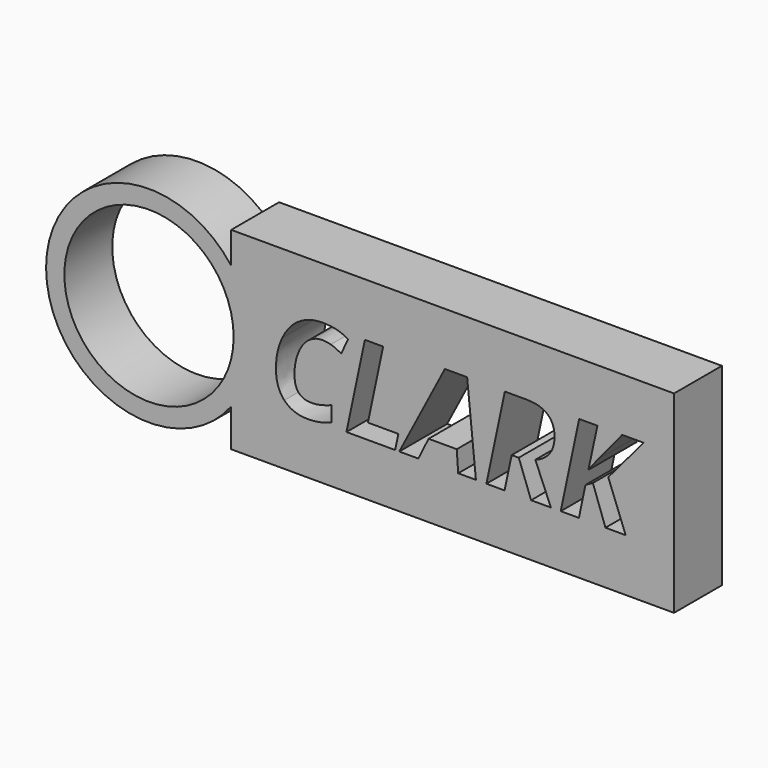
from build123d import *

# Parameters (mm, degrees)
F0_R     = 35.3591127091
F1_DEPTH = 25


with BuildPart() as f1:
    # F0 (on Front) → F1 (new body)
    with BuildSketch(Plane.XZ):
        with BuildLine():
            Line((61.9367249054, 34.8669122506), (-123.0632750946, 34.8669122506))
            Line((-123.0632750946, 34.8669122506), (-123.0632750946, 21.6819903858))
            ThreePointArc((-123.0632750946, 21.6819903858), (-116.6274794012, 9.4492653106), (-114.4056740389, -4.193410743))
            ThreePointArc((-114.4056740389, -4.193410743), (-116.6274794012, -17.8360867967), (-123.0632750946, -30.0688118719))
            Line((-123.0632750946, -30.0688118719), (-123.0632750946, -45.8291395163))
            Line((-123.0632750946, -45.8291395163), (61.9367249054, -45.8291395163))
            Line((61.9367249054, -45.8291395163), (61.9367249054, 34.8669122506))
        make_face()
        with BuildLine():
            add(Edge.make_bspline(
                [(-81.4851504642, 6.2619487625), (-83.2026240645, 6.7321619524), (-84.9001733771, 6.7321619524)],
                knots=[0, 0, 0, 1, 1, 1], degree=2))
            add(Edge.make_bspline(
                [(-84.9001733771, 6.7321619524), (-88.1836959912, 6.7321619524), (-90.8137019684, 4.7158240365)],
                knots=[0, 0, 0, 1, 1, 1], degree=2))
            add(Edge.make_bspline(
                [(-90.8137019684, 4.7158240365), (-93.4437079457, 2.6994861206), (-95.0376509623, -1.2216137001)],
                knots=[0, 0, 0, 1, 1, 1], degree=2))
            add(Edge.make_bspline(
                [(-95.0376509623, -1.2216137001), (-96.6315939788, -5.1427135208), (-96.6315939788, -9.6535722576)],
                knots=[0, 0, 0, 1, 1, 1], degree=2))
            add(Edge.make_bspline(
                [(-96.6315939788, -9.6535722576), (-96.6315939788, -13.8137635308), (-94.9260749511, -15.8301014467)],
                knots=[0, 0, 0, 1, 1, 1], degree=2))
            add(Edge.make_bspline(
                [(-94.9260749511, -15.8301014467), (-93.2205559234, -17.8464393626), (-89.4827595496, -17.8464393626)],
                knots=[0, 0, 0, 1, 1, 1], degree=2))
            add(Edge.make_bspline(
                [(-89.4827595496, -17.8464393626), (-85.8485694719, -17.8464393626), (-81.0667404223, -15.9257380277)],
                knots=[0, 0, 0, 1, 1, 1], degree=2))
            Line((-81.0667404223, -15.9257380277), (-81.0667404223, -22.4051163899))
            add(Edge.make_bspline(
                [(-81.0667404223, -22.4051163899), (-86.0159334887, -24.3258177248), (-91.0288842757, -24.3258177248)],
                knots=[0, 0, 0, 1, 1, 1], degree=2))
            add(Edge.make_bspline(
                [(-91.0288842757, -24.3258177248), (-97.3488683362, -24.3258177248), (-100.8635126877, -20.5999759237)],
                knots=[0, 0, 0, 1, 1, 1], degree=2))
            add(Edge.make_bspline(
                [(-100.8635126877, -20.5999759237), (-104.3781570392, -16.8741341225), (-104.3781570392, -10.0520580117)],
                knots=[0, 0, 0, 1, 1, 1], degree=2))
            add(Edge.make_bspline(
                [(-104.3781570392, -10.0520580117), (-104.3781570392, -3.524861359), (-101.7879996373, 1.9662723329)],
                knots=[0, 0, 0, 1, 1, 1], degree=2))
            add(Edge.make_bspline(
                [(-101.7879996373, 1.9662723329), (-99.1978422354, 7.4574060249), (-94.8623172304, 10.3105640245)],
                knots=[0, 0, 0, 1, 1, 1], degree=2))
            add(Edge.make_bspline(
                [(-94.8623172304, 10.3105640245), (-90.5267922255, 13.1637220241), (-84.9001733771, 13.1637220241)],
                knots=[0, 0, 0, 1, 1, 1], degree=2))
            add(Edge.make_bspline(
                [(-84.9001733771, 13.1637220241), (-81.7840147798, 13.1637220241), (-79.3691911097, 12.6018571108)],
                knots=[0, 0, 0, 1, 1, 1], degree=2))
            add(Edge.make_bspline(
                [(-79.3691911097, 12.6018571108), (-76.9543674396, 12.0399921975), (-74.188876306, 10.549655477)],
                knots=[0, 0, 0, 1, 1, 1], degree=2))
            Line((-74.188876306, 10.549655477), (-77.1297011715, 4.3173382823))
            add(Edge.make_bspline(
                [(-77.1297011715, 4.3173382823), (-79.7676768638, 5.7917355726), (-81.4851504642, 6.2619487625)],
                knots=[0, 0, 0, 1, 1, 1], degree=2))
        make_face(mode=Mode.SUBTRACT)
        Polygon((-54.5594680573, -23.8237256746), (-74.9061506634, -23.8237256746), (-67.2153756086, 12.5899025382), (-59.5883582745, 12.5899025382), (-65.9641303406, -17.4479536085), (-53.2125862083, -17.4479536085), align=None, mode=Mode.SUBTRACT)
        Polygon((-28.2354991392, -23.8237256746), (-28.8332277704, -15.1526756647), (-40.6124666626, -15.1526756647), (-44.892203662, -23.8237256746), (-52.8619187447, -23.8237256746), (-33.7903905518, 12.7413271247), (-24.4977027654, 12.7413271247), (-20.8396035425, -23.8237256746), align=None, mode=Mode.SUBTRACT)
        with BuildLine():
            Line((-2.9236840366, -9.8528151347), (-5.8884180473, -9.8528151347))
            Line((-5.8884180473, -9.8528151347), (-8.8531520581, -23.8237256746))
            Line((-8.8531520581, -23.8237256746), (-16.4482905319, -23.8237256746))
            Line((-16.4482905319, -23.8237256746), (-8.7575154771, 12.5899025382))
            Line((-8.7575154771, 12.5899025382), (0.1845048457, 12.5899025382))
            add(Edge.make_bspline(
                [(0.1845048457, 12.5899025382), (6.0900637219, 12.5899025382), (9.0547977327, 10.0475634268)],
                knots=[0, 0, 0, 1, 1, 1], degree=2))
            add(Edge.make_bspline(
                [(9.0547977327, 10.0475634268), (12.0195317435, 7.5052243154), (12.0195317435, 2.6038495396)],
                knots=[0, 0, 0, 1, 1, 1], degree=2))
            add(Edge.make_bspline(
                [(12.0195317435, 2.6038495396), (12.0195317435, -1.3331897113), (9.9513906795, -4.1584537081)],
                knots=[0, 0, 0, 1, 1, 1], degree=2))
            add(Edge.make_bspline(
                [(9.9513906795, -4.1584537081), (7.8832496155, -6.9837177049), (3.9940286552, -8.3545086991)],
                knots=[0, 0, 0, 1, 1, 1], degree=2))
            Line((3.9940286552, -8.3545086991), (10.4973161627, -23.8237256746))
            Line((10.4973161627, -23.8237256746), (2.2247519068, -23.8237256746))
            Line((2.2247519068, -23.8237256746), (-2.9236840366, -9.8528151347))
        make_face(mode=Mode.SUBTRACT)
        Polygon((34.4542797012, -4.8478340628), (41.7067204265, -23.8237256746), (33.2827315841, -23.8237256746), (28.0306893446, -9.0797527717), (24.9145307472, -10.8251203748), (22.2048276191, -23.8237256746), (14.6096891453, -23.8237256746), (22.3004642001, 12.5899025382), (29.9274815343, 12.5899025382), (26.14186687, -4.8956523532), (30.0709364057, 0.2129350148), (40.2562322814, 12.5899025382), (49.2540406098, 12.5899025382), align=None, mode=Mode.SUBTRACT)
        with BuildLine():
            ThreePointArc((-114.4056740389, -4.193410743), (-116.6274794012, 9.4492653106), (-123.0632750946, 21.6819903858))
            ThreePointArc((-123.0632750946, 21.6819903858), (-200.3983681841, -4.193410743), (-123.0632750946, -30.0688118719))
            ThreePointArc((-123.0632750946, -30.0688118719), (-116.6274794012, -17.8360867967), (-114.4056740389, -4.193410743))
        make_face()
        with Locations((-157.4020211115, -4.193410743)):
            Circle(F0_R, mode=Mode.SUBTRACT)
    extrude(amount=F1_DEPTH)


solid = f1.part
